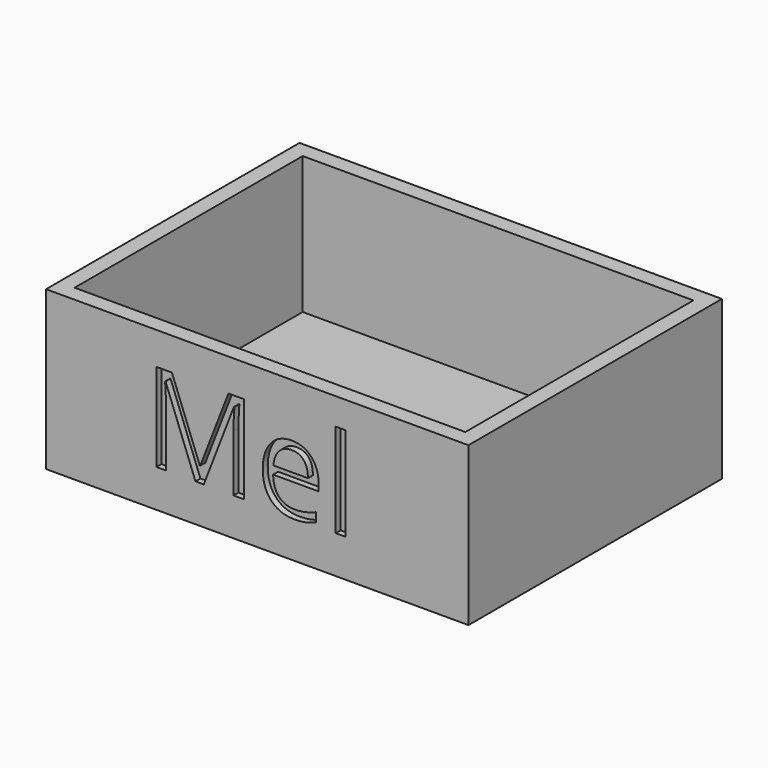
from build123d import *

# Parameters (mm, degrees)
F0_W         = 101.6
F0_H         = 76.2
F1_DEPTH     = 38.1
F2_W         = 93.98
F2_H         = 68.58
F3_DEPTH     = 33.02
F4_TEXT_SIZE = 29.7018339754
F5_DEPTH     = 1.5


# Not quite as in the source:
# - Text() gives the source's letters only with a copy of the font that has no kerning and outlines rounded to 1/6400 em; it was checked with that copy


with BuildPart() as f1:
    # F0 (on Top) → F1 (new body)
    with BuildSketch(Plane.XY):
        Rectangle(F0_W, F0_H)
    extrude(amount=F1_DEPTH)

    # F2 (on face) → F3 (cut)
    with BuildSketch(Plane.XY.offset(38.1)):
        Rectangle(F2_W, F2_H)
    extrude(amount=-F3_DEPTH, mode=Mode.SUBTRACT)

    # F4 (on face) → F5 (cut)
    with BuildSketch(Plane.XZ.offset(38.1)):
        with Locations((-27.1651344374, 9.0798148885)):
            Text('Mel', F4_TEXT_SIZE, font='Open Sans', text_align=(TextAlign.LEFT, TextAlign.BOTTOM))
    extrude(amount=-F5_DEPTH, mode=Mode.SUBTRACT)


solid = f1.part
